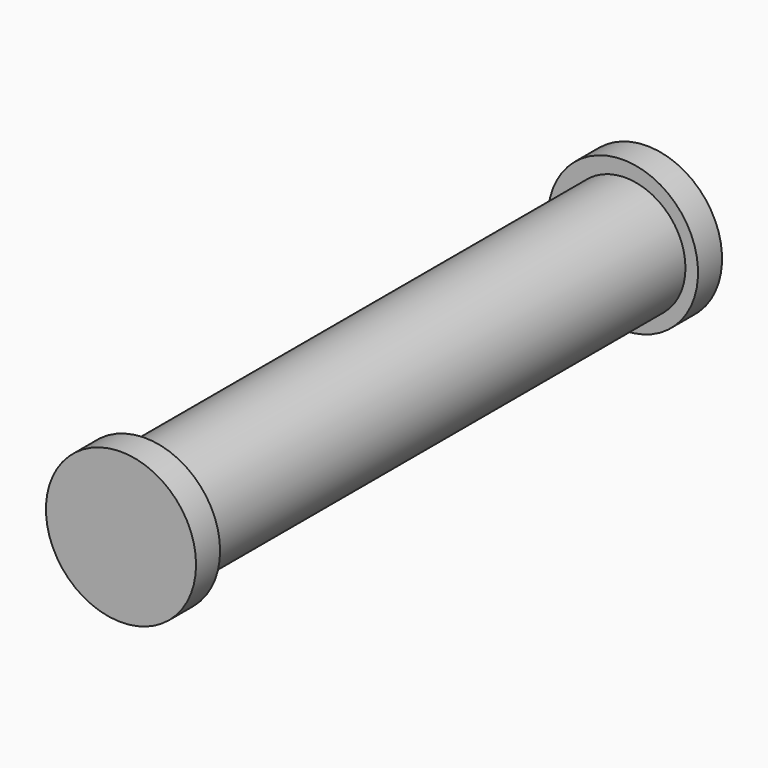
from build123d import *

# Parameters (mm, degrees)
F0_R     = 4
F1_DEPTH = 40
F2_R     = 5
F2_R_2   = 4
F3_DEPTH = 2
F4_R     = 5
F4_R_2   = 4
F5_DEPTH = 2


with BuildPart() as f1:
    # F0 (on Front) → F1 (new body)
    with BuildSketch(Plane.XZ):
        Circle(F0_R)
    extrude(amount=F1_DEPTH)

    # F2 (on face) → F3 (join)
    with BuildSketch(Plane.XZ.offset(40)):
        Circle(F2_R)
        Circle(F2_R_2, mode=Mode.SUBTRACT)
        Circle(F2_R_2)
    extrude(amount=F3_DEPTH)

    # F4 (on face) → F5 (join)
    with BuildSketch(Plane(origin=(0, 0, 0), x_dir=(-1, 0, 0), z_dir=(0, 1, 0))):
        with Locations((0.1622709678, 0)):
            Circle(F4_R)
        Circle(F4_R_2, mode=Mode.SUBTRACT)
        Circle(F4_R_2)
    extrude(amount=F5_DEPTH)


solid = f1.part
